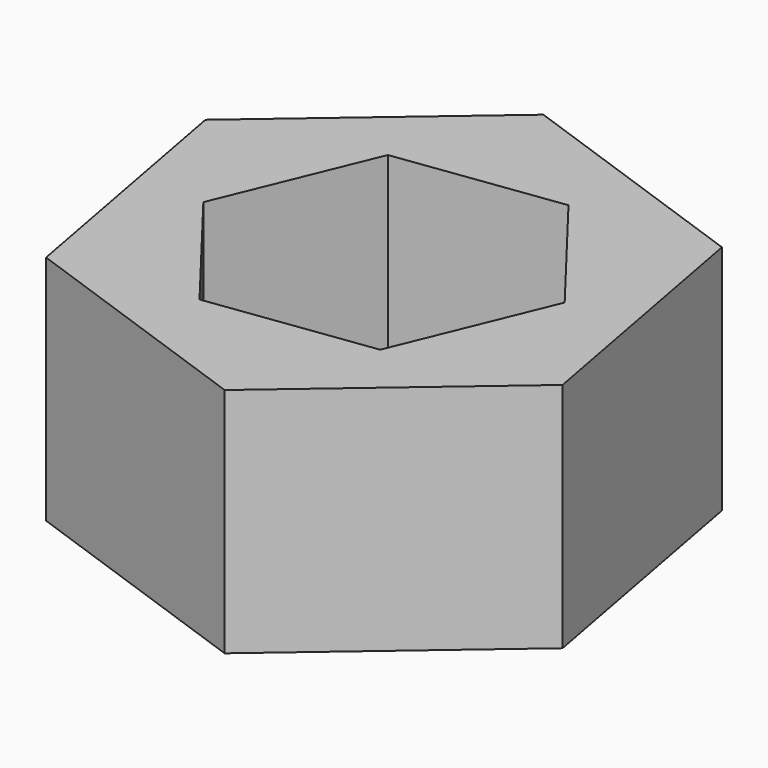
from build123d import *

# Parameters (mm, degrees)
F1_DEPTH = 50.8
F3_DEPTH = 50.8


# Not quite as in the source:
# - a feature names something its author has since deleted; it is built from what else it names


with BuildPart() as f1:
    # F0 (on Top) → F1 (new body)
    with BuildSketch(Plane.XY):
        Polygon((10.580912179, -56.8864221716), (54.5555428205, -19.2798723436), (43.9746306415, 37.606549828), (-10.580912179, 56.8864221716), (-54.5555428205, 19.2798723436), (-43.9746306415, -37.606549828), align=None)
    extrude(amount=F1_DEPTH)

    # F2 (on face) → F3 (cut)
    with BuildSketch(Plane.XY.offset(50.8)):
        Polygon((22.0264125762, -28.5840980822), (35.7677613716, 4.7833838041), (13.7413487954, 33.3674818864), (-22.0264125762, 28.5840980822), (-35.7677613716, -4.7833838041), (-13.7413487954, -33.3674818864), align=None)
    extrude(amount=-F3_DEPTH, mode=Mode.SUBTRACT)


solid = f1.part
